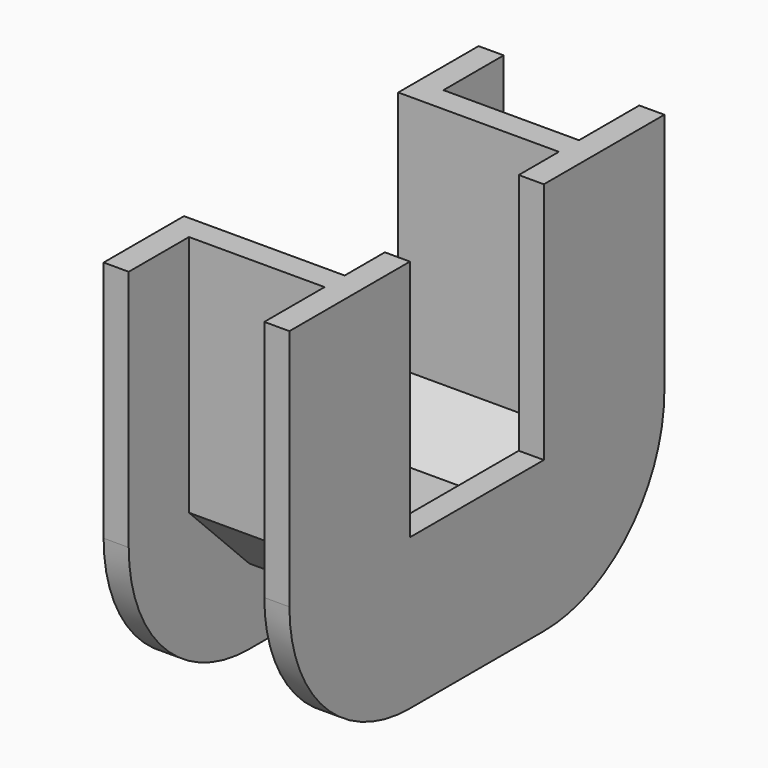
from build123d import *

# Parameters (mm, degrees)
F2_DEPTH = 11.1
F4_DEPTH = 3
F6_DEPTH = 3


# Not quite as in the source:
# - a pattern or mirror of a feature is missing from the dataset's text; its kind, count and spacing are read off the source's solid


with BuildPart() as f2:
    # F1 (on Right) → F2 (new body, symmetric)
    with BuildSketch(Plane.YZ):
        Polygon((-16, 0), (-19, 0), (-19, -29), (-10, -38), (-6, -38), (6, -38), (10.1178772148, -38), (19, -29), (19, 0), (16, 0), (16, -29), (10, -35), (0, -35), (-10, -35), (-16, -29), align=None)
    extrude(amount=F2_DEPTH, both=True)

    # F3 (on face) → F4 (join)
    with BuildSketch(Plane.YZ.offset(11.1)):
        with BuildLine():
            Line((-28, 0), (-28, -29))
            ThreePointArc((-28, -29), (-22.7279220614, -41.7279220614), (-10, -47))
            Line((-10, -47), (10, -47))
            ThreePointArc((10, -47), (22.7279220614, -41.7279220614), (28, -29))
            Line((28, -29), (28, 0))
            Line((28, 0), (19, 0))
            Line((19, 0), (19, -29))
            Line((19, -29), (10.1178772148, -38))
            Line((10.1178772148, -38), (-10, -38))
            Line((-10, -38), (-19, -29))
            Line((-19, -29), (-19, 0))
            Line((-19, 0), (-28, 0))
        make_face()
    f4 = extrude(amount=-F4_DEPTH)

    # F4_copies: F4 across plane
    add(f4.mirror(Plane(origin=(0, 0, 0), x_dir=(0, 0, -1), z_dir=(-1, 0, 0))))

    # F5 (on face) → F6 (join)
    with BuildSketch(Plane.YZ.offset(11.1)):
        Polygon((10, 0), (10, -29), (-10, -29), (-10, 0), (-16, 0), (-16, -29), (-10, -35), (0, -35), (10, -35), (16, -29), (16, 0), align=None)
    extrude(amount=-F6_DEPTH)


solid = f2.part
